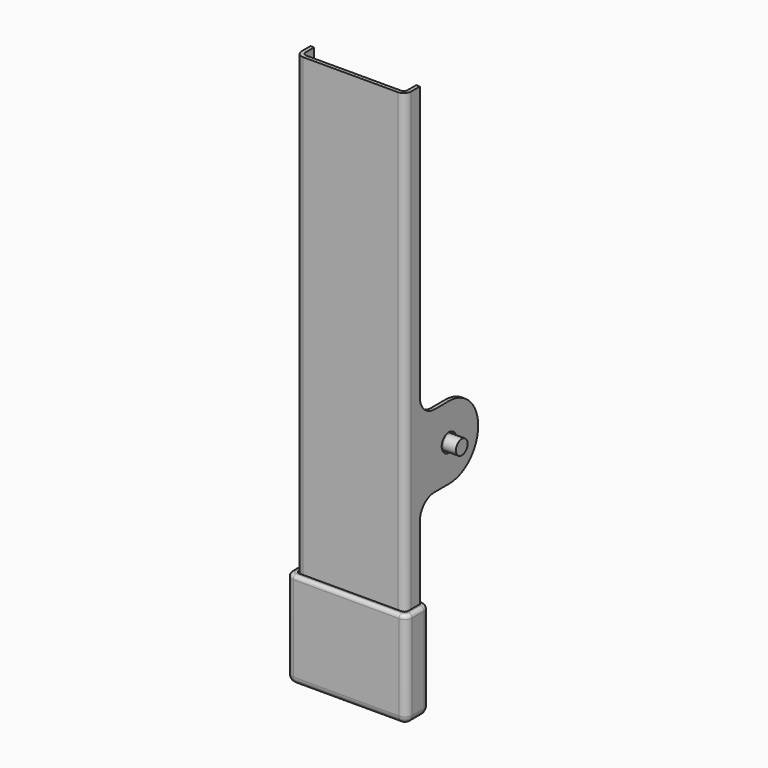
from build123d import *

# Parameters (mm, degrees)
F1_DEPTH       = 150
F2_R           = 2.5
F3_DEPTH       = 1
F4_R           = 5
F5_R           = 2.5
F6_DEPTH       = 1
F7_R           = 5
F10_R          = 2
F11_DEPTH      = 31.5
F11_DEPTH_BACK = 3.5
F13_DEPTH      = 25
F15_DEPTH      = 1.5
F16_R          = 2
F17_R          = 1


with BuildPart() as f1:
    # F0 (on Top) → F1 (new body)
    with BuildSketch(Plane.XY):
        with BuildLine():
            ThreePointArc((0, 2), (0.5857864376, 0.5857864376), (2, 0))
            Line((2, 0), (28, 0))
            ThreePointArc((28, 0), (29.4142135624, 0.5857864376), (30, 2))
            Line((30, 2), (30, 5))
            Line((30, 5), (29, 5))
            Line((29, 5), (29, 2))
            ThreePointArc((29, 2), (28.7071067812, 1.2928932188), (28, 1))
            Line((28, 1), (2, 1))
            ThreePointArc((2, 1), (1.2928932188, 1.2928932188), (1, 2))
            Line((1, 2), (1, 5))
            Line((1, 5), (0, 5))
            Line((0, 5), (0, 2))
        make_face()
    extrude(amount=F1_DEPTH)

    # F2 (on face) → F3 (join)
    with BuildSketch(Plane(origin=(0, 0, 0), x_dir=(0, -1, 0), z_dir=(-1, 0, 0))):
        with BuildLine():
            Line((-15, 50), (-5, 50))
            Line((-5, 50), (-5, 70))
            Line((-5, 70), (-15, 70))
            ThreePointArc((-15, 70), (-22.0710678119, 67.0710678119), (-25, 60))
            ThreePointArc((-25, 60), (-22.0710678119, 52.9289321881), (-15, 50))
        make_face()
        with Locations((-15, 60)):
            Circle(F2_R, mode=Mode.SUBTRACT)
    extrude(amount=-F3_DEPTH)

    # F4
    f4_edges = [f1.edges().sort_by_distance(p)[0] for p in [
        (0.5, 5, 50),
        (0.5, 5, 70),
    ]]
    fillet(f4_edges, radius=F4_R)

    # F5 (on face) → F6 (join)
    with BuildSketch(Plane.YZ.offset(30)):
        with BuildLine():
            Line((15, 70), (5, 70))
            Line((5, 70), (5, 50))
            Line((5, 50), (15, 50))
            ThreePointArc((15, 50), (22.0710678119, 52.9289321881), (25, 60))
            ThreePointArc((25, 60), (22.0710678119, 67.0710678119), (15, 70))
        make_face()
        with Locations((15, 60)):
            Circle(F5_R, mode=Mode.SUBTRACT)
    extrude(amount=-F6_DEPTH)

    # F7
    f7_edges = [f1.edges().sort_by_distance(p)[0] for p in [
        (29.5, 5, 70),
        (29.5, 5, 50),
    ]]
    fillet(f7_edges, radius=F7_R)


with BuildPart() as f8_1:
    # F8: copy of F1
    add(f1.part.moved(Location((0, 75, 0))))


with BuildPart() as f11:
    # F10 (on face) → F11 (new body, two sides)
    with BuildSketch(Plane.YZ.offset(30)) as f11_sk:
        with Locations((15, 60)):
            Circle(F10_R)
    extrude(amount=-F11_DEPTH)
    extrude(f11_sk.sketch, amount=F11_DEPTH_BACK)


with BuildPart() as f13:
    # F12 (on face) → F13 (new body)
    with BuildSketch(Plane(origin=(0, 0, 0), x_dir=(1, 0, 0), z_dir=(0, 0, -1))):
        with BuildLine():
            Line((31.5, -4.5), (31.5, -0.5))
            ThreePointArc((31.5, -0.5), (30.9142135624, 0.9142135624), (29.5, 1.5))
            Line((29.5, 1.5), (0.5, 1.5))
            ThreePointArc((0.5, 1.5), (-0.9142135624, 0.9142135624), (-1.5, -0.5))
            Line((-1.5, -0.5), (-1.5, -4.5))
            ThreePointArc((-1.5, -4.5), (-0.9142135624, -5.9142135624), (0.5, -6.5))
            Line((0.5, -6.5), (29.5, -6.5))
            ThreePointArc((29.5, -6.5), (30.9142135624, -5.9142135624), (31.5, -4.5))
        make_face()
        with BuildLine():
            ThreePointArc((0, -1), (0.2928932188, -0.2928932188), (1, 0))
            Line((1, 0), (2, 0))
            Line((2, 0), (28, 0))
            Line((28, 0), (29, 0))
            ThreePointArc((29, 0), (29.7071067812, -0.2928932188), (30, -1))
            Line((30, -1), (30, -2))
            Line((30, -2), (30, -5))
            Line((30, -5), (29, -5))
            Line((29, -5), (1, -5))
            Line((1, -5), (0, -5))
            Line((0, -5), (0, -2))
            Line((0, -2), (0, -1))
        make_face(mode=Mode.SUBTRACT)
    extrude(amount=-F13_DEPTH)

    # F14 (on face) → F15 (join)
    with BuildSketch(Plane(origin=(0, 0, 0), x_dir=(1, 0, 0), z_dir=(0, 0, -1))):
        with BuildLine():
            Line((29.5, 1.5), (0.5, 1.5))
            ThreePointArc((0.5, 1.5), (-0.9142135624, 0.9142135624), (-1.5, -0.5))
            Line((-1.5, -0.5), (-1.5, -4.5))
            ThreePointArc((-1.5, -4.5), (-0.9142135624, -5.9142135624), (0.5, -6.5))
            Line((0.5, -6.5), (29.5, -6.5))
            ThreePointArc((29.5, -6.5), (30.9142135624, -5.9142135624), (31.5, -4.5))
            Line((31.5, -4.5), (31.5, -0.5))
            ThreePointArc((31.5, -0.5), (30.9142135624, 0.9142135624), (29.5, 1.5))
        make_face()
    extrude(amount=F15_DEPTH)

    # F16
    f16_edges = [f13.edges().sort_by_distance(p)[0] for p in [
        (15, -1.5, -1.5),
        (-0.914214, 5.914214, -1.5),
        (-1.5, 2.5, -1.5),
        (-0.914214, -0.914214, -1.5),
        (30.914214, -0.914214, -1.5),
        (31.5, 2.5, -1.5),
        (30.914214, 5.914214, -1.5),
        (15, 6.5, -1.5),
    ]]
    fillet(f16_edges, radius=F16_R)

    # F17
    f17_edges = [f13.edges().sort_by_distance(p)[0] for p in [
        (15, -1.5, 25),
        (-0.914214, 5.914214, 25),
        (15, 6.5, 25),
        (30.914214, 5.914214, 25),
        (31.5, 2.5, 25),
        (30.914214, -0.914214, 25),
        (-0.914214, -0.914214, 25),
        (-1.5, 2.5, 25),
    ]]
    fillet(f17_edges, radius=F17_R)


solid = Compound([f1.part, f11.part, f13.part])
